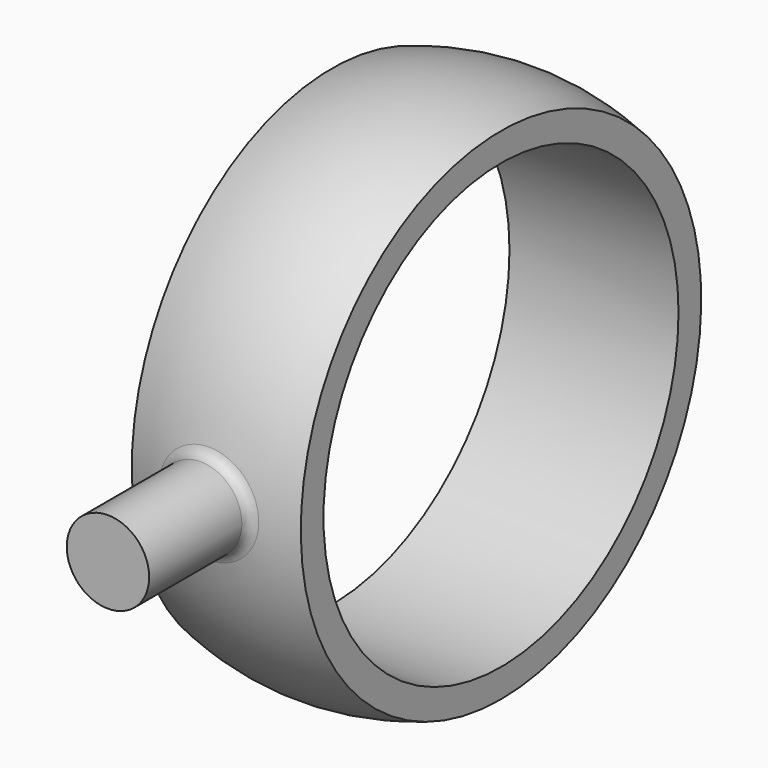
from build123d import *

# Parameters (mm, degrees)
F2_W      = 21.7011459378
F2_H      = 87.9080442688
F2_W_2    = 24.2758599693
F2_H_2    = 94.1609184015
F3_DEPTH  = 30
F4_R      = 20
F5_DEPTH  = 15
F6_R      = 21
F7_DEPTH  = 30
F9_R      = 3.9
F10_DEPTH = 1.5
F11_DEPTH = 10
F13_R     = 1


with BuildPart() as f1:
    # F0 (on Front) → F1 (revolve)
    with BuildSketch(Plane.XZ):
        with BuildLine():
            Line((25, 0), (21, 0))
            ThreePointArc((21, 0), (0, -21), (-21, 0))
            Line((-21, 0), (-25, 0))
            ThreePointArc((-25, 0), (0, -25), (25, 0))
        make_face()
    revolve(axis=Axis((0, 0, 0), (1, 0, 0)))

    # F2 (on Front) → F3 (cut, symmetric)
    with BuildSketch(Plane.XZ):
        with Locations((18.8505729689, -0.3834927207)):
            Rectangle(F2_W, F2_H)
        with Locations((-20.1379299847, -2.4064816535)):
            Rectangle(F2_W_2, F2_H_2)
    extrude(amount=F3_DEPTH, both=True, mode=Mode.SUBTRACT)

    # F4 (on face) → F5 (cut)
    with BuildSketch(Plane.YZ.offset(8)):
        Circle(F4_R)
    extrude(amount=-F5_DEPTH, mode=Mode.SUBTRACT)

    # F6 (on face) → F7 (cut, symmetric)
    with BuildSketch(Plane.YZ.offset(8)):
        Circle(F6_R)
    extrude(amount=F7_DEPTH, both=True, mode=Mode.SUBTRACT)


with BuildPart() as f10:
    # F9 (on offset) → F10 (new body, symmetric)
    with BuildSketch(Plane.XZ.offset(25)):
        Circle(F9_R)
    extrude(amount=F10_DEPTH, both=True)

    # F11 (add): a face of the model
    f11_faces = [f10.faces().sort_by_distance(p)[0] for p in [
        (0, -26.5, 0),
    ]]
    extrude(f11_faces, amount=F11_DEPTH)

    # F12: union F1
    add(f1.part)

    # F13
    f13_edges = [f10.edges().sort_by_distance(p)[0] for p in [
        (-3.9, -24.693926, 0),
    ]]
    fillet(f13_edges, radius=F13_R)


solid = f10.part
